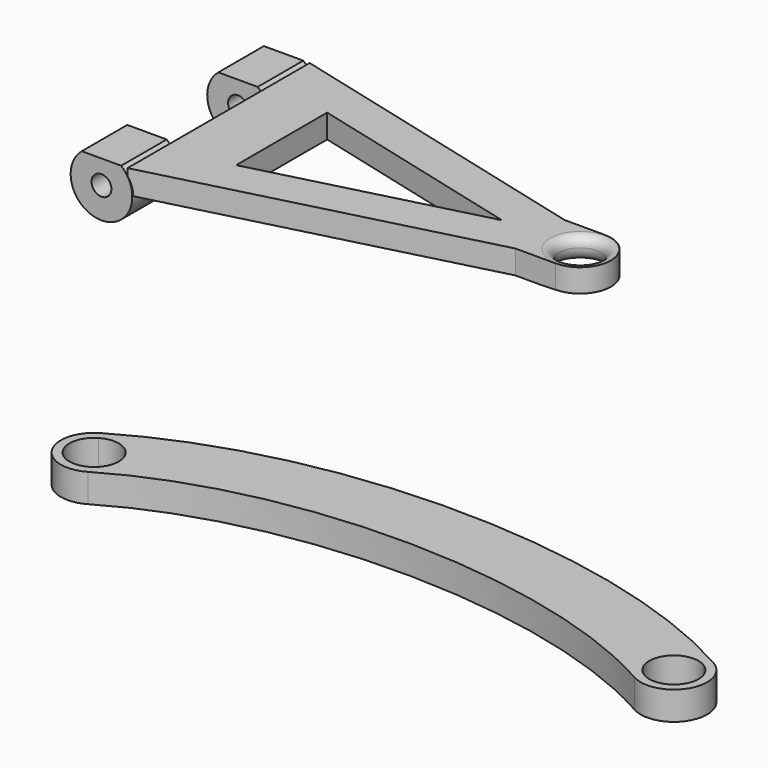
from build123d import *

# Parameters (mm, degrees)
F0_R     = 2.15
F1_DEPTH = 2.5
F0_W     = 2.2
F0_H     = 6
F4_DEPTH = 25
F5_R     = 1
F7_DEPTH = 3


# Not quite as in the source:
# - a fillet or chamfer that OpenCascade refuses, or shapes differently, is made with other operations: its cross-section is extruded or revolved along the edge and cut away or added
# - ends of sketch curves that miss each other by under 0.0002 mm in the source are joined


with BuildPart() as f1:
    # F0 (on Top) → F1 (new body)
    with BuildSketch(Plane.XY):
        with BuildLine():
            Line((-21.4300396313, 18), (-21.4300396313, 12))
            Line((-21.4300396313, 12), (-21.4300396313, 0))
            Line((-21.4300396313, 0), (-21.4300396313, -6))
            Line((-21.4300396313, -6), (12.458564648, 2.75))
            Line((12.458564648, 2.75), (16.6866835368, 2.75))
            ThreePointArc((16.6866835368, 2.75), (19.9366835368, 6), (16.6866835368, 9.25))
            Line((16.6866835368, 9.25), (12.458564648, 9.25))
            Line((12.458564648, 9.25), (-21.4300396313, 18))
        make_face()
        Polygon((-14.7793354293, 0), (-14.7793354293, 12), (8.458564648, 6), align=None, mode=Mode.SUBTRACT)
        with Locations((16.6866835368, 6)):
            Circle(F0_R, mode=Mode.SUBTRACT)
    extrude(amount=F1_DEPTH)

    # F0 (on Top) → F2 (revolve)
    with BuildSketch(Plane.XY):
        with Locations((-26.3300396313, 15)):
            Rectangle(F0_W, F0_H)
        with Locations((-26.3300396313, -3)):
            Rectangle(F0_W, F0_H)
    revolve(axis=Axis((-24.1800396313, 6, 0), (0, -1, 0)))

    # F3 (on face) → F4 (cut)
    with BuildSketch(Plane.XY.offset(2.5)):
        Polygon((-32.1821644902, -8.1532467157), (-17.6776833832, -8.1532467157), (-17.6776833832, -5.0311457828), (-21.4300396313, -6), (-21.4300396313, 18), (-17.6776833832, 17.0311457828), (-17.6776833832, 19.4846000522), (-32.1821644902, 19.4846000522), align=None)
    extrude(amount=F4_DEPTH, mode=Mode.SUBTRACT)

    # F5
    f5_edges = [f1.edges().sort_by_distance(p)[0] for p in [
        (14.536684, 6, 2.5),
    ]]
    fillet(f5_edges, radius=F5_R)

    # F8: fillet of radius 1.5 on 1 edges, made by hand

    # F8_s1 → F8_t2 (revolve, cut)
    with BuildSketch(Plane.XZ.offset(-6)):
        with BuildLine():
            ThreePointArc((18.8366835368, 1.5), (19.276023365, 0.4393398282), (20.3366835368, 0))
            Line((20.3366835368, 0), (18.8366835368, 0))
            Line((18.8366835368, 0), (18.8366835368, 1.5))
        make_face()
    revolve(axis=Axis((16.6866835368, 6, 0), (0, 0, 1)), mode=Mode.SUBTRACT)


with BuildPart() as f7:
    # F6 (on Top) → F7 (new body)
    with BuildSketch(Plane.XY):
        with BuildLine():
            Line((10.0186065005, -50.2990549731), (10.4777156403, -51.0731472142))
            add(Edge.make_bspline(
                [(10.4777156403, -51.0731472142), (25.9556712089, -41.8932711085), (52.4891549721, -42.5315449635), (68.4777156403, -51.5755629086)],
                knots=[0, 0, 0, 0, 58.0021760069, 58.0021760069, 58.0021760069, 58.0021760069], degree=3))
            Line((68.4777156403, -51.5755629086), (68.9208272734, -50.7922034249))
            ThreePointArc((68.9208272734, -50.7922034249), (67.9378890383, -47.2490646433), (71.4810278199, -46.2661264081))
            Line((71.4810278199, -46.2661264081), (71.9241399568, -45.4827660336))
            add(Edge.make_bspline(
                [(6.9068662528, -45.0524289032), (9.2342901511, -43.6720487272), (14.1852496401, -41.3479130597), (22.2369017105, -39.0014371496), (30.7031876351, -37.6850142792), (39.3799195161, -37.3354743879), (48.0612605365, -37.9192740739), (56.5400497137, -39.4258205208), (64.6099834157, -41.8693760457), (69.5798404734, -44.1567000395), (71.9241399568, -45.4827660336)],
                knots=[0, 0, 0, 0, 0.125, 0.25, 0.375, 0.5, 0.625, 0.75, 0.875, 1, 1, 1, 1], degree=3))
            Line((6.9068662528, -45.0524289032), (7.3659759147, -45.8265220246))
            ThreePointArc((7.3659759147, -45.8265220246), (9.9790662926, -45.8035386497), (11.2922912076, -48.0627884988))
            ThreePointArc((11.2922912076, -48.0627884988), (10.9515410567, -49.3495635838), (10.0186065005, -50.2990549731))
        make_face()
        with BuildLine():
            ThreePointArc((6.9068667749, -45.0524297835), (5.6819324923, -49.8482129316), (10.4777156403, -51.0731472142))
            Line((10.4777156403, -51.0731472142), (10.0186065005, -50.2990549731))
            ThreePointArc((10.0186065005, -50.2990549731), (6.4560247334, -49.3891037917), (7.3659759147, -45.8265220246))
            Line((7.3659759147, -45.8265220246), (6.9068667749, -45.0524297835))
        make_face()
        with BuildLine():
            Line((68.9208272734, -50.7922034249), (68.4777156403, -51.5755629086))
            ThreePointArc((68.4777156403, -51.5755629086), (73.2473255387, -50.2523768228), (71.9241394529, -45.4827669245))
            Line((71.9241394529, -45.4827669245), (71.4810278199, -46.2661264081))
            ThreePointArc((71.4810278199, -46.2661264081), (72.4468416935, -47.2192528413), (72.8009275466, -48.5291649165))
            ThreePointArc((72.8009275466, -48.5291649165), (71.5108396218, -50.7750790634), (68.9208272734, -50.7922034249))
        make_face()
    extrude(amount=F7_DEPTH)


solid = Compound([f1.part, f7.part])
